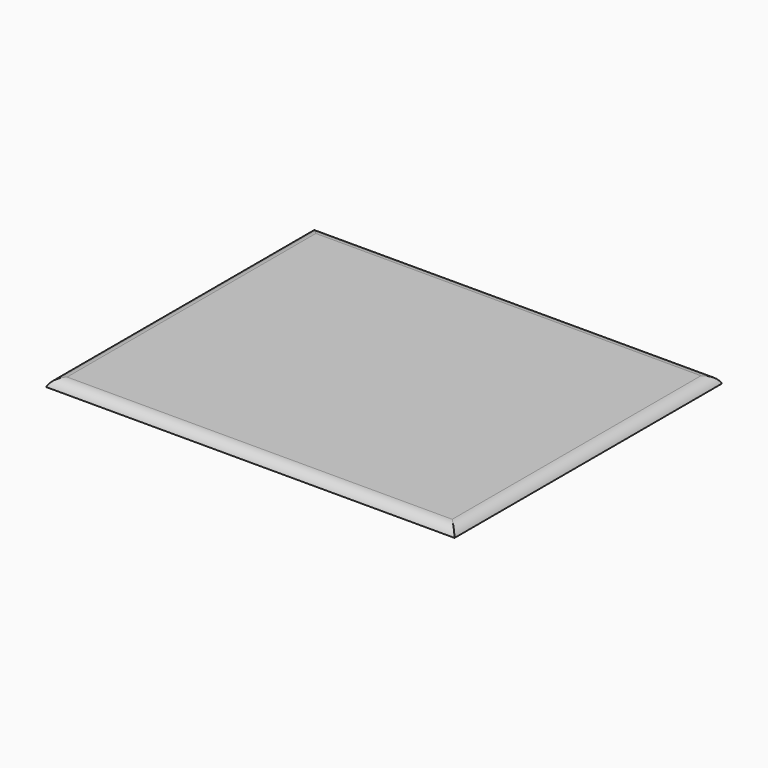
from build123d import *

# Parameters (mm, degrees)
F0_W        = 165
F0_H        = 135
F1_DEPTH    = 3.175
F2_T1_DEPTH = 158.5464301965
F2_T3_DEPTH = 188.5464301965


# Not quite as in the source:
# - a fillet or chamfer that OpenCascade refuses, or shapes differently, is made with other operations: its cross-section is extruded or revolved along the edge and cut away or added


with BuildPart() as f1:
    # F0 (on Top) → F1 (new body)
    with BuildSketch(Plane.XY):
        Rectangle(F0_W, F0_H)
    extrude(amount=F1_DEPTH)

    # F2: fillet of radius 5.08 on 4 edges, made by hand

    # F2_s2 → F2_t1 (cut)
    with BuildSketch(Plane.XZ.offset(-79.2732150983)):
        with BuildLine():
            ThreePointArc((-82.5, 0), (-80.6305202921, 2.3071134838), (-77.7907139607, 3.175))
            Line((-77.7907139607, 3.175), (-82.5, 3.175))
            Line((-82.5, 3.175), (-82.5, 0))
        make_face()
        with BuildLine():
            ThreePointArc((82.5, 0), (80.6305202921, 2.3071134838), (77.7907139607, 3.175))
            Line((77.7907139607, 3.175), (82.5, 3.175))
            Line((82.5, 3.175), (82.5, 0))
        make_face()
    extrude(amount=F2_T1_DEPTH, mode=Mode.SUBTRACT)

    # F2_s4 → F2_t3 (cut)
    with BuildSketch(Plane.YZ.offset(-94.2732150983)):
        with BuildLine():
            ThreePointArc((-67.5, 0), (-65.6305202921, 2.3071134838), (-62.7907139607, 3.175))
            Line((-62.7907139607, 3.175), (-67.5, 3.175))
            Line((-67.5, 3.175), (-67.5, 0))
        make_face()
        with BuildLine():
            ThreePointArc((67.5, 0), (65.6305202921, 2.3071134838), (62.7907139607, 3.175))
            Line((62.7907139607, 3.175), (67.5, 3.175))
            Line((67.5, 3.175), (67.5, 0))
        make_face()
    extrude(amount=F2_T3_DEPTH, mode=Mode.SUBTRACT)


solid = f1.part
